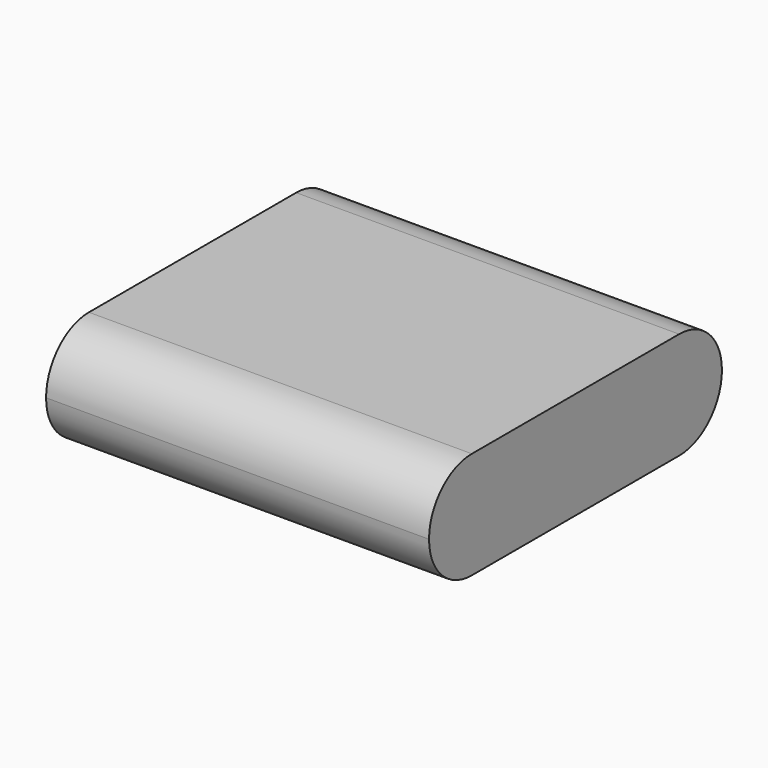
from build123d import *

# Parameters (mm, degrees)
F0_W     = 65
F0_H     = 19
F1_DEPTH = 34
F2_R     = 9.49999


# Not quite as in the source:
# - a fillet or chamfer is up to 0.001 mm smaller than in the source, because OpenCascade refuses the exact size


with BuildPart() as f1:
    # F0 (on Right) → F1 (new body, symmetric)
    with BuildSketch(Plane.YZ):
        Rectangle(F0_W, F0_H)
    extrude(amount=F1_DEPTH, both=True)

    # F2 (radius 9.5 in the source; OpenCascade refuses exactly that, so slightly less here)
    f2_edges = [f1.edges().sort_by_distance(p)[0] for p in [
        (0, -32.5, 9.5),
        (0, -32.5, -9.5),
        (0, 32.5, 9.5),
        (0, 32.5, -9.5),
    ]]
    fillet(f2_edges, radius=F2_R)


solid = f1.part
